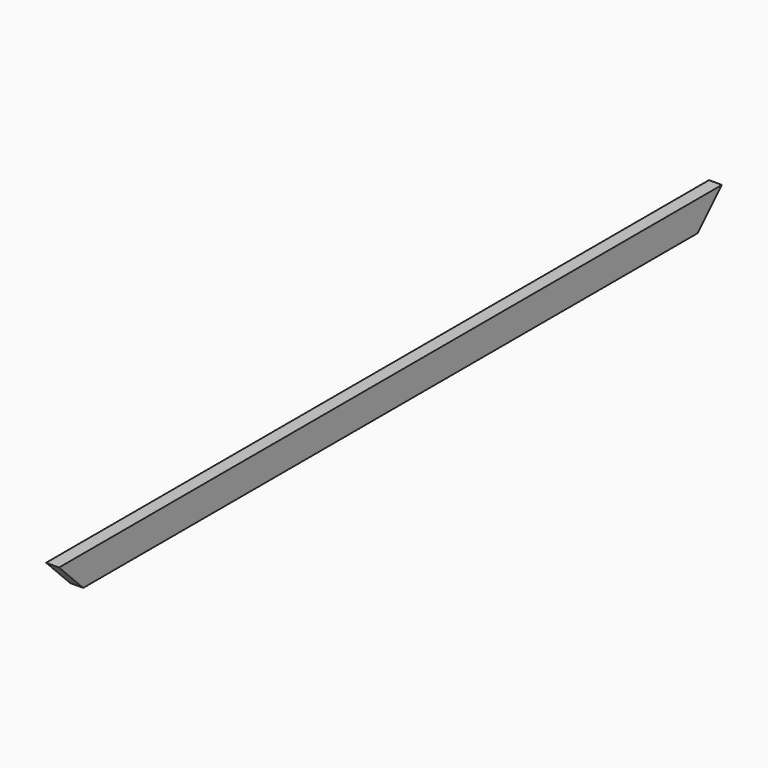
from build123d import *

# Parameters (mm, degrees)
F0_W     = 38.1
F0_H     = 88.9
F1_DEPTH = 1219.2
F2_SIZE2 = 88.89999
F2_SIZE  = 88.89999
F3_SIZE2 = 88.89999
F3_SIZE  = 88.89999


# Not quite as in the source:
# - a fillet or chamfer is up to 0.001 mm smaller than in the source, because OpenCascade refuses the exact size


with BuildPart() as f1:
    # F0 (on Front) → F1 (new body, symmetric)
    with BuildSketch(Plane.XZ):
        Rectangle(F0_W, F0_H)
    extrude(amount=F1_DEPTH, both=True)

    # F2 (size 88.9 and 88.9 in the source; OpenCascade refuses exactly that, so slightly less here)
    f2_edges = [f1.edges().sort_by_distance(p)[0] for p in [
        (0, -1219.2, -44.45),
    ]]
    chamfer(f2_edges, length=F2_SIZE, length2=F2_SIZE2)

    # F3 (size 88.9 and 88.9 in the source; OpenCascade refuses exactly that, so slightly less here)
    f3_edges = [f1.edges().sort_by_distance(p)[0] for p in [
        (0, 1219.2, -44.45),
    ]]
    chamfer(f3_edges, length=F3_SIZE, length2=F3_SIZE2)


solid = f1.part
